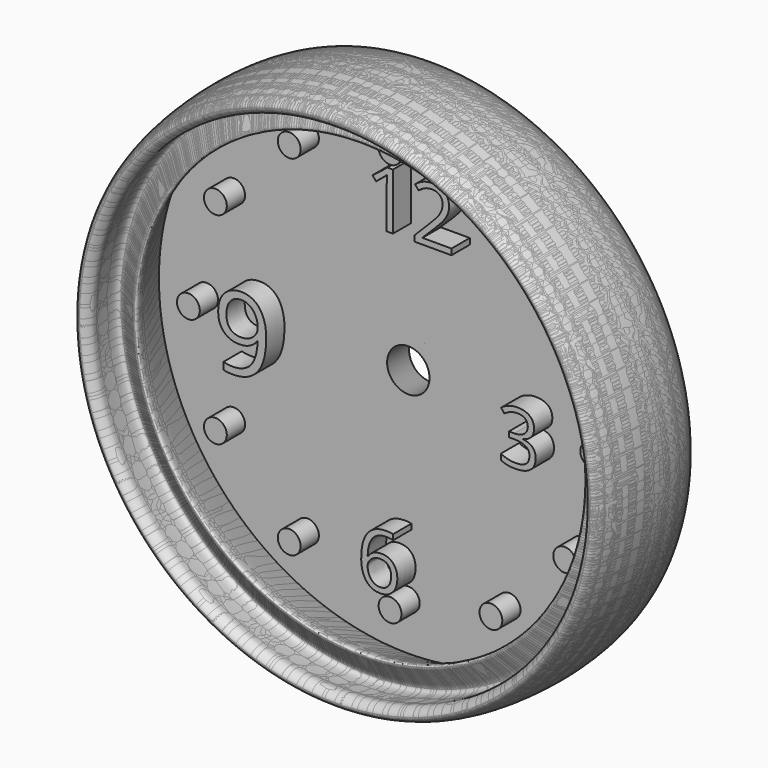
from build123d import *

# Parameters (mm, degrees)
F2_R           = 5
F3_DEPTH       = 10
F4_COUNT       = 12
F5_TEXT_SIZE   = 34.6090437637
F5_TEXT_SIZE_2 = 32.6500416526
F5_TEXT_SIZE_3 = 33.9560417665
F5_TEXT_SIZE_4 = 45.0570563165
F6_DEPTH       = 10


# Not quite as in the source:
# - Text() gives the source's letters only with a copy of the font that has no kerning and outlines rounded to 1/6400 em; it was checked with that copy


with BuildPart() as f1:
    # F0 (on Right) → F1 (revolve)
    with BuildSketch(Plane.YZ):
        with BuildLine():
            Line((-36.7224402726, 9.2939501628), (-24.7224402726, 9.2939501628))
            Line((-24.7224402726, 9.2939501628), (-24.7224402726, 89.2939501628))
            add(Edge.make_bspline(
                [(-36.7224402726, 109.2939501628), (-49.973362158, 102.6057615719), (-71.6411618059, 91.6692900079), (-51.6664488071, 113.0851296508), (-70.6826959506, 109.1230825072), (-74.4167962796, 108.3106571853), (-83.3198083751, 116.7800585061), (-10.9554480463, 123.3536669494), (-20.7357903256, 99.1569736824), (-24.7224402726, 89.2939501628)],
                knots=[0, 0, 0, 0, 0.18614408, 0.3043812851, 0.4246930683, 0.5036349194, 0.573346428, 0.8260880456, 1, 1, 1, 1], degree=3))
            Line((-36.7224402726, 109.2939501628), (-36.7224402726, 9.2939501628))
        make_face()
    revolve(axis=Axis((0, -30.6020341814, 0), (0, -1, 0)))

    # F2 (on face) → F3 (join)
    with BuildSketch(Plane.XZ.offset(36.7224402726)):
        with Locations((0, 88.3065909147)):
            Circle(F2_R)
    extrude(amount=F3_DEPTH)


with BuildPart() as f4_1:
    # F4: instance of F1
    add(f1.part.rotate(Axis((0, -36.7224402726, 0), (0, -1, 0)), 1 * 360 / F4_COUNT))


with BuildPart() as f4_2:
    # F4: instance of F1
    add(f1.part.rotate(Axis((0, -36.7224402726, 0), (0, -1, 0)), 2 * 360 / F4_COUNT))


with BuildPart() as f4_3:
    # F4: instance of F1
    add(f1.part.rotate(Axis((0, -36.7224402726, 0), (0, -1, 0)), 3 * 360 / F4_COUNT))


with BuildPart() as f4_4:
    # F4: instance of F1
    add(f1.part.rotate(Axis((0, -36.7224402726, 0), (0, -1, 0)), 4 * 360 / F4_COUNT))


with BuildPart() as f4_5:
    # F4: instance of F1
    add(f1.part.rotate(Axis((0, -36.7224402726, 0), (0, -1, 0)), 5 * 360 / F4_COUNT))


with BuildPart() as f4_6:
    # F4: instance of F1
    add(f1.part.rotate(Axis((0, -36.7224402726, 0), (0, -1, 0)), 6 * 360 / F4_COUNT))


with BuildPart() as f4_7:
    # F4: instance of F1
    add(f1.part.rotate(Axis((0, -36.7224402726, 0), (0, -1, 0)), 7 * 360 / F4_COUNT))


with BuildPart() as f4_8:
    # F4: instance of F1
    add(f1.part.rotate(Axis((0, -36.7224402726, 0), (0, -1, 0)), 8 * 360 / F4_COUNT))


with BuildPart() as f4_9:
    # F4: instance of F1
    add(f1.part.rotate(Axis((0, -36.7224402726, 0), (0, -1, 0)), 9 * 360 / F4_COUNT))


with BuildPart() as f4_10:
    # F4: instance of F1
    add(f1.part.rotate(Axis((0, -36.7224402726, 0), (0, -1, 0)), 10 * 360 / F4_COUNT))


with BuildPart() as f4_11:
    # F4: instance of F1
    add(f1.part.rotate(Axis((0, -36.7224402726, 0), (0, -1, 0)), 11 * 360 / F4_COUNT))


with BuildPart() as f6:
    # F5 (on face) → F6 (new body)
    with BuildSketch(Plane.XZ.offset(36.7224402726)):
        with Locations((-10.8136925846, 57.1245104074)):
            Text('12', F5_TEXT_SIZE, font='Open Sans', text_align=(TextAlign.LEFT, TextAlign.BOTTOM))
        with Locations((47.0160543919, -15.7503802329)):
            Text('3', F5_TEXT_SIZE_2, font='Open Sans', text_align=(TextAlign.LEFT, TextAlign.BOTTOM))
        with Locations((-14.574976638, -82.9833447933)):
            Text('6', F5_TEXT_SIZE_3, font='Open Sans', text_align=(TextAlign.LEFT, TextAlign.BOTTOM))
        with Locations((-77.576495707, -19.5116642863)):
            Text('9', F5_TEXT_SIZE_4, font='Open Sans', text_align=(TextAlign.LEFT, TextAlign.BOTTOM))
    extrude(amount=F6_DEPTH)


solid = Compound([f1.part, f4_1.part, f4_2.part, f4_3.part, f4_4.part, f4_5.part, f4_6.part, f4_7.part, f4_8.part, f4_9.part, f4_10.part, f4_11.part, f6.part])
